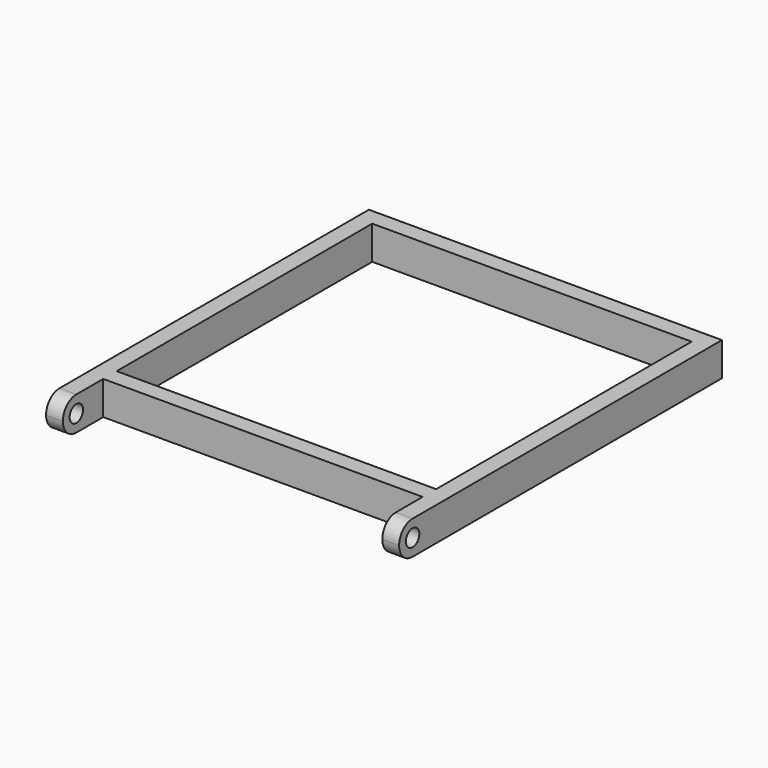
from build123d import *

# Parameters (mm, degrees)
F0_W     = 5
F0_H     = 15
F1_DEPTH = 10
F2_R     = 2.5
F3_DEPTH = 105.001
F4_R     = 4.99999
F5_W     = 95
F5_H     = 95
F6_DEPTH = 10.001


# Not quite as in the source:
# - a fillet or chamfer is up to 0.001 mm smaller than in the source, because OpenCascade refuses the exact size


with BuildPart() as f1:
    # F0 (on Top) → F1 (new body)
    with BuildSketch(Plane.XY):
        Polygon((52.5, 52.5), (-52.5, 52.5), (-52.5, -52.5), (-47.5, -52.5), (47.5, -52.5), (52.5, -52.5), align=None)
        with Locations((-50, -60)):
            Rectangle(F0_W, F0_H)
        with Locations((50, -60)):
            Rectangle(F0_W, F0_H)
    extrude(amount=F1_DEPTH)

    # F2 (on face) → F3 (cut, through all)
    with BuildSketch(Plane.YZ.offset(52.5)):
        with Locations((-62.5, 5)):
            Circle(F2_R)
    extrude(amount=-F3_DEPTH, mode=Mode.SUBTRACT)

    # F4 (radius 5 in the source; OpenCascade refuses exactly that, so slightly less here)
    f4_edges = [f1.edges().sort_by_distance(p)[0] for p in [
        (-50, -67.5, 10),
        (-50, -67.5, 0),
        (50, -67.5, 10),
        (50, -67.5, 0),
    ]]
    fillet(f4_edges, radius=F4_R)

    # F5 (on face) → F6 (cut, through all)
    with BuildSketch(Plane.XY.offset(10)):
        Rectangle(F5_W, F5_H)
    extrude(amount=-F6_DEPTH, mode=Mode.SUBTRACT)


solid = f1.part
